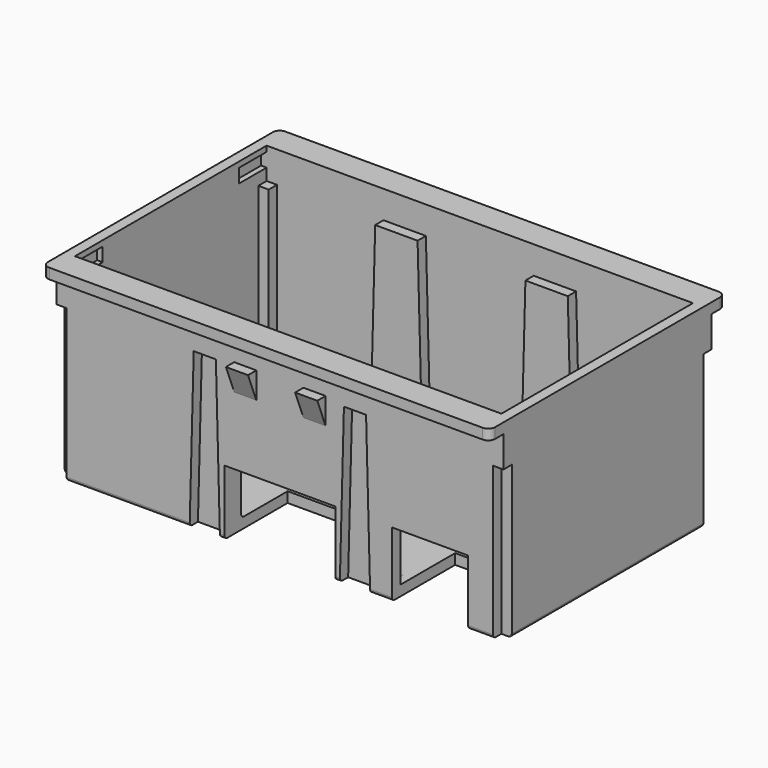
from build123d import *

# Parameters (mm, degrees)
F0_W      = 64.6
F0_H      = 37.6
F1_DEPTH  = 28
F3_DEPTH  = 1.5
F4_W      = 1.5
F4_H      = 1.5
F5_DEPTH  = 22
F6_T      = -1.5
F7_W      = 64.6
F7_H      = 2.5
F8_DEPTH  = 1.5
F9_W      = 5
F9_H      = 2
F10_DEPTH = 31.6
F11_W     = 3.2
F11_H     = 3.8
F12_DEPTH = 1.5
F14_DEPTH = 38.901
F15_W     = 16
F15_H     = 11.4
F15_W_2   = 11
F16_DEPTH = 9.4
F17_R     = 1
F18_R     = 0.5


# Not quite as in the source:
# - two fillets or chamfers of one size are made in one step
# - a pattern or mirror of a feature is missing from the dataset's text; its kind, count and spacing are read off the source's solid


with BuildPart() as f1:
    # F0 (on Top) → F1 (new body)
    with BuildSketch(Plane.XY):
        Rectangle(F0_W, F0_H)
    extrude(amount=F1_DEPTH)

    # F2 (on face) → F3 (cut)
    with BuildSketch(Plane.XZ.offset(18.8)):
        Polygon((-13.0391832353, 0), (-8.6608167647, 0), (-9.25, 22.5), (-12.45, 22.5), align=None)
        Polygon((12.45, 22.5), (9.25, 22.5), (8.6608167647, 0), (13.0391832353, 0), align=None)
    f3 = extrude(amount=-F3_DEPTH, mode=Mode.SUBTRACT)

    # F3_copies: F3 across plane
    add(f3.mirror(Plane.ZX), mode=Mode.SUBTRACT)

    # F4 (on face) → F5 (cut)
    with BuildSketch(Plane(origin=(0, 0, 0), x_dir=(1, 0, 0), z_dir=(0, 0, -1))):
        with Locations((-31.55, 18.05)):
            Rectangle(F4_W, F4_H)
        with Locations((31.55, 18.05)):
            Rectangle(F4_W, F4_H)
        with Locations((31.55, -18.05)):
            Rectangle(F4_W, F4_H)
        with Locations((-31.55, -18.05)):
            Rectangle(F4_W, F4_H)
    extrude(amount=-F5_DEPTH, mode=Mode.SUBTRACT)

    # F6
    f6_openings = [f1.faces().sort_by_distance(p)[0] for p in [
        (0, 0, 28),
    ]]
    offset(amount=F6_T, openings=f6_openings, kind=Kind.INTERSECTION)

    # F7 (on face) → F8 (join)
    with BuildSketch(Plane.XY.offset(28)):
        with Locations((0, -20.05)):
            Rectangle(F7_W, F7_H)
        with Locations((0, 20.05)):
            Rectangle(F7_W, F7_H)
    extrude(amount=-F8_DEPTH)

    # F9 (on Right) → F10 (cut, symmetric)
    with BuildSketch(Plane.YZ):
        with Locations((-14.8, 26.2)):
            Rectangle(F9_W, F9_H)
        with Locations((14.8, 26.2)):
            Rectangle(F9_W, F9_H)
    extrude(amount=F10_DEPTH, both=True, mode=Mode.SUBTRACT)

    # F11 (on face) → F12 (join)
    with BuildSketch(Plane.XZ.offset(18.8)):
        with Locations((-5, 21.1)):
            Rectangle(F11_W, F11_H)
        with Locations((5, 21.1)):
            Rectangle(F11_W, F11_H)
    f12 = extrude(amount=F12_DEPTH)

    # F12_copies: F12 across plane
    add(f12.mirror(Plane.ZX))

    # F13 (on face) → F14 (cut, through all)
    with BuildSketch(Plane.YZ.offset(6.6)):
        Polygon((-18.8, 19.2), (-20.3, 23), (-20.3, 19.2), align=None)
    f14 = extrude(amount=-F14_DEPTH, mode=Mode.SUBTRACT)

    # F14_copies: F14 across plane
    add(f14.mirror(Plane.ZX), mode=Mode.SUBTRACT)

    # F15 (on face) → F16 (cut)
    with BuildSketch(Plane(origin=(0, 0, 0), x_dir=(1, 0, 0), z_dir=(0, 0, -1))):
        with Locations((0, 13.1)):
            Rectangle(F15_W, F15_H)
        with Locations((21.7, 13.1)):
            Rectangle(F15_W_2, F15_H)
    extrude(amount=-F16_DEPTH, mode=Mode.SUBTRACT)

    # F17
    f17_edges = [f1.edges().sort_by_distance(p)[0] for p in [
        (32.3, -21.3, 27.25),
        (32.3, 21.3, 27.25),
        (-32.3, -21.3, 27.25),
        (-32.3, 21.3, 27.25),
    ]]
    fillet(f17_edges, radius=F17_R)

    # F18
    f18_edges = [f1.edges().sort_by_distance(p)[0] for p in [
        (32.3, 0, 0),
        (29, -18.8, 0),
        (14.619592, -18.8, 0),
        (-8.330408, -18.8, 0),
        (-21.919592, -18.8, 0),
        (-32.3, 0, 0),
        (0, 18.8, 0),
        (8.330408, -18.8, 0),
        (-21.919592, 18.8, 0),
        (21.919592, 18.8, 0),
        (30.8, 0, 1.5),
        (-21.900209, -17.3, 1.5),
        (28.25, -17.3, 1.5),
        (-30.8, 0, 1.5),
        (-21.900209, 17.3, 1.5),
        (0, 17.3, 1.5),
        (21.900209, 17.3, 1.5),
        (29.3, -16.55, 1.5),
        (14.500419, -16.55, 1.5),
        (11.250209, -15.8, 1.5),
        (-11.250209, -15.8, 1.5),
        (-14.500419, -16.55, 1.5),
        (-29.3, -16.55, 1.5),
        (-30.05, -15.8, 1.5),
        (-30.05, 15.8, 1.5),
        (-29.3, 16.55, 1.5),
        (-14.500419, 16.55, 1.5),
        (-10.85, 15.8, 1.5),
        (-7.199581, 16.55, 1.5),
        (7.199581, 16.55, 1.5),
        (10.85, 15.8, 1.5),
        (14.500419, 16.55, 1.5),
        (29.3, 16.55, 1.5),
        (30.05, 15.8, 1.5),
        (30.05, -15.8, 1.5),
    ]]
    fillet(f18_edges, radius=F18_R)


solid = f1.part
